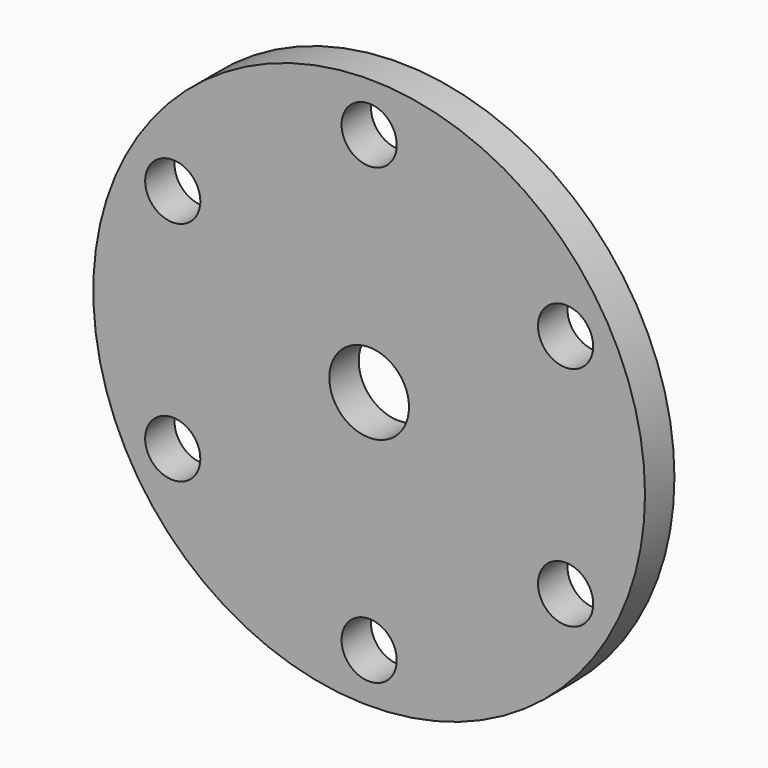
from build123d import *

# Parameters (mm, degrees)
F0_R            = 45
F0_R_2          = 6.5
F1_DEPTH        = 3
F2_R            = 4.5
F3_DEPTH        = 25
F3_COPIES_COUNT = 6


# Not quite as in the source:
# - a pattern or mirror of a feature is missing from the dataset's text; its kind, count and spacing are read off the source's solid


with BuildPart() as f1:
    # F0 (on Front) → F1 (new body, symmetric)
    with BuildSketch(Plane.XZ):
        Circle(F0_R)
        Circle(F0_R_2, mode=Mode.SUBTRACT)
    extrude(amount=F1_DEPTH, both=True)

    # F2 (on face) → F3 (cut)
    with BuildSketch(Plane.XZ.offset(3)):
        with Locations((0, 37)):
            Circle(F2_R)
    f3 = extrude(amount=-F3_DEPTH, mode=Mode.SUBTRACT)

    # F3_copies: F3 ×6 about axis
    f3_copies_axis = Axis((0, 0, 0), (0, 1, 0))
    for i in range(1, F3_COPIES_COUNT):
        add(f3.rotate(f3_copies_axis, i * 360 / F3_COPIES_COUNT), mode=Mode.SUBTRACT)


solid = f1.part
